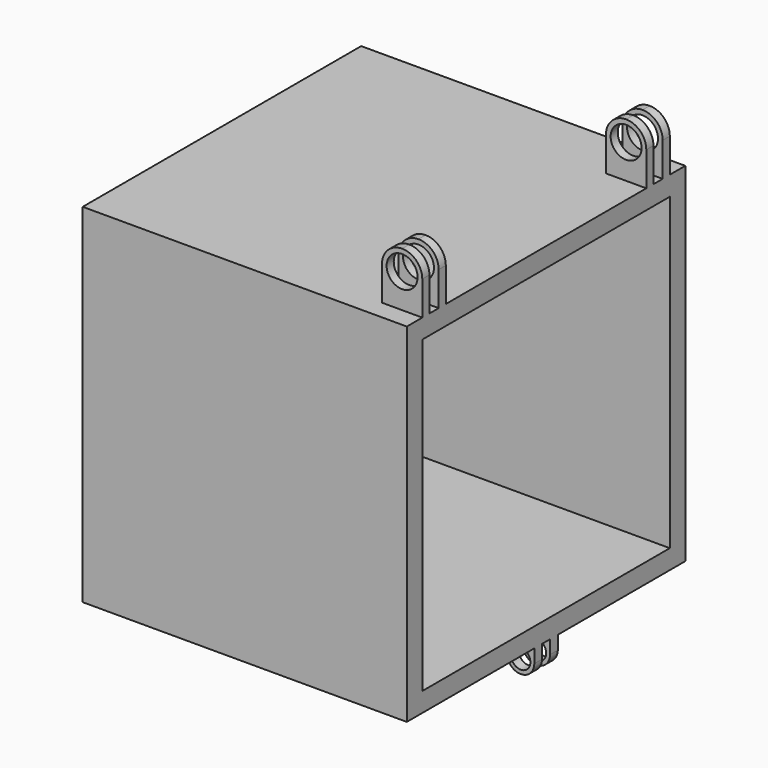
from build123d import *

# Parameters (mm, degrees)
F0_W      = 114.3
F0_H      = 114.3
F0_W_2    = 101.6
F0_H_2    = 101.6
F1_DEPTH  = 106.426
F2_W      = 114.3
F2_H      = 114.3
F3_DEPTH  = 6.35
F4_W      = 13.2588
F4_H      = 9.652
F5_DEPTH  = 17.78
F6_W      = 3.81
F6_H      = 17.78
F7_DEPTH  = 106.427
F8_R      = 6.62939
F9_R      = 5.08
F10_DEPTH = 25.4
F11_W     = 8.89
F11_H     = 3.175
F12_DEPTH = 8.89
F13_R     = 4.44499
F14_R     = 3.175
F15_DEPTH = 25.4


# Not quite as in the source:
# - a fillet or chamfer is up to 0.001 mm smaller than in the source, because OpenCascade refuses the exact size
# - a pattern or mirror of a feature is missing from the dataset's text; its kind, count and spacing are read off the source's solid


with BuildPart() as f1:
    # F0 (on Right) → F1 (new body)
    with BuildSketch(Plane.YZ):
        Rectangle(F0_W, F0_H)
        Rectangle(F0_W_2, F0_H_2, mode=Mode.SUBTRACT)
    extrude(amount=F1_DEPTH)

    # F2 (on Right) → F3 (join)
    with BuildSketch(Plane.YZ):
        Rectangle(F2_W, F2_H)
    extrude(amount=F3_DEPTH)

    # F4 (on face) → F5 (join)
    with BuildSketch(Plane.XY.offset(57.15)):
        with Locations((99.7966, 45.974)):
            Rectangle(F4_W, F4_H)
    f5 = extrude(amount=F5_DEPTH)

    # F5_copies: F5 across plane
    add(f5.mirror(Plane(origin=(0, 2e-06, 0), x_dir=(0, 0, -1), z_dir=(0, -1, 0))))

    # F6 (on face) → F7 (cut, through all)
    with BuildSketch(Plane.YZ.offset(106.426)):
        with Locations((45.974, 66.04)):
            Rectangle(F6_W, F6_H)
    f7 = extrude(amount=-F7_DEPTH, mode=Mode.SUBTRACT)

    # F7_copies: F7 across plane
    add(f7.mirror(Plane(origin=(0, 3e-06, 0), x_dir=(0, 0, -1), z_dir=(0, -1, 0))), mode=Mode.SUBTRACT)

    # F8 (radius 6.6294 in the source; OpenCascade refuses exactly that, so slightly less here)
    f8_edges = [f1.edges().sort_by_distance(p)[0] for p in [
        (106.426, 49.3395, 74.93),
        (106.426, 42.6085, 74.93),
        (93.1672, 49.3395, 74.93),
        (93.1672, 42.6085, 74.93),
        (93.1672, -49.339495, 74.93),
        (106.426, -49.339495, 74.93),
        (93.1672, -42.608495, 74.93),
        (106.426, -42.608495, 74.93),
    ]]
    fillet(f8_edges, radius=F8_R)

    # F9 (on face) → F10 (cut)
    with BuildSketch(Plane(origin=(0, 50.8, 0), x_dir=(-1, 0, 0), z_dir=(0, 1, 0))):
        with Locations((-99.7966, 68.3006)):
            Circle(F9_R)
    f10 = extrude(amount=-F10_DEPTH, mode=Mode.SUBTRACT)

    # F10_copies: F10 across plane
    add(f10.mirror(Plane(origin=(0, 0, 0), x_dir=(0, 0, -1), z_dir=(0, -1, 0))), mode=Mode.SUBTRACT)

    # F11 (on face) → F12 (join)
    with BuildSketch(Plane(origin=(0, 0, -57.15), x_dir=(1, 0, 0), z_dir=(0, 0, -1))):
        with Locations((101.981, 3.2385)):
            Rectangle(F11_W, F11_H)
        with Locations((101.981, -3.2385)):
            Rectangle(F11_W, F11_H)
    extrude(amount=F12_DEPTH)

    # F13 (radius 4.445 in the source; OpenCascade refuses exactly that, so slightly less here)
    f13_edges = [f1.edges().sort_by_distance(p)[0] for p in [
        (97.536, -3.2385, -66.04),
        (97.536, 3.2385, -66.04),
        (106.426, 3.2385, -66.04),
        (106.426, -3.2385, -66.04),
    ]]
    fillet(f13_edges, radius=F13_R)

    # F14 (on face) → F15 (cut)
    with BuildSketch(Plane.XZ.offset(4.826)):
        with Locations((101.981, -61.595)):
            Circle(F14_R)
    extrude(amount=-F15_DEPTH, mode=Mode.SUBTRACT)


solid = f1.part
